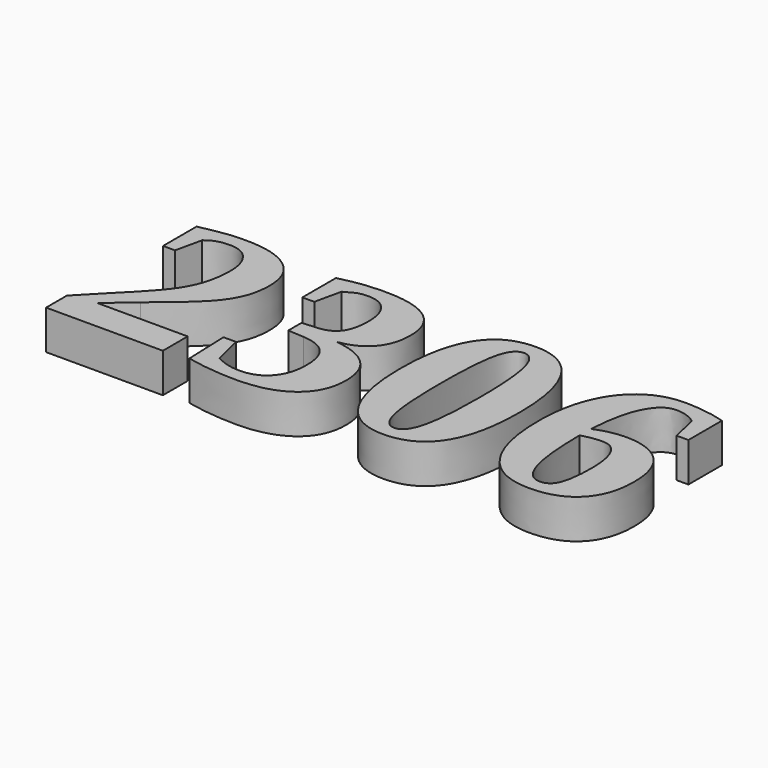
from build123d import *

# Parameters (mm, degrees)
F0_TEXT_SIZE = 86.1111111111
F1_DEPTH     = 12


# Not quite as in the source:
# - Text() gives the source's letters only with a copy of the font that has no kerning and outlines rounded to 1/6400 em; it was checked with that copy


with BuildPart() as f1:
    # F0 (on Top) → F1 (new body)
    with BuildSketch(Plane.XY):
        with Locations((-87.5440538194, -30.6075908738)):
            Text('2306', F0_TEXT_SIZE, font='Tinos', font_style=FontStyle.BOLD, text_align=(TextAlign.LEFT, TextAlign.BOTTOM))
    extrude(amount=F1_DEPTH)


solid = f1.part
